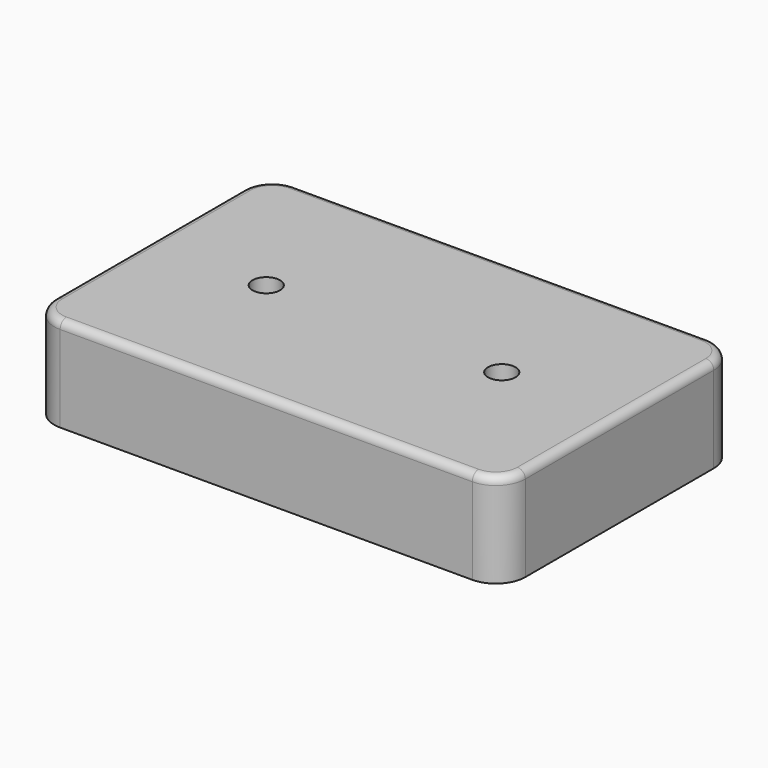
from build123d import *

# Parameters (mm, degrees)
F0_W         = 120
F0_H         = 75
F1_DEPTH     = 4
F2_W         = 120
F2_H         = 75
F3_DEPTH     = 20
F4_R         = 2
F5_T1_DEPTH  = 42.75
F5_T4_ANGLE  = 90
F5_T6_ANGLE  = 90
F5_T8_ANGLE  = 90
F5_T10_ANGLE = 90
F6_R         = 3.5
F7_DEPTH     = 25
F8_R         = 1.7577503979
F8_R_2       = 1.75
F9_DEPTH     = 10


# Not quite as in the source:
# - a fillet or chamfer that OpenCascade refuses, or shapes differently, is made with other operations: its cross-section is extruded or revolved along the edge and cut away or added


with BuildPart() as f1:
    # F0 (on Top) → F1 (new body)
    with BuildSketch(Plane.XY):
        Rectangle(F0_W, F0_H)
    extrude(amount=F1_DEPTH)

    # F2 (on face) → F3 (join)
    with BuildSketch(Plane(origin=(0, 0, 0), x_dir=(1, 0, 0), z_dir=(0, 0, -1))):
        Rectangle(F2_W, F2_H)
        Polygon((54.339364171, -27.5), (50, -27.5), (50, -31.3459709287), (-50, -31.3459709287), (-50, -27.5), (-54.5065030456, -27.5), (-54.5065030456, 27.5), (-50, 27.5), (-50, 32.2239883244), (50, 32.2239883244), (50, 27.5), (54.339364171, 27.5), align=None, mode=Mode.SUBTRACT)
    extrude(amount=F3_DEPTH)

    # F4
    f4_edges = [f1.edges().sort_by_distance(p)[0] for p in [
        (60, 0, 4),
        (0, -37.5, 4),
        (-60, 0, 4),
        (0, 37.5, 4),
    ]]
    fillet(f4_edges, radius=F4_R)

    # F5: fillet of radius 7.5 on 4 edges, made by hand

    # F5_s2 → F5_t1 (cut)
    with BuildSketch(Plane.XY.offset(-38.75)):
        with BuildLine():
            ThreePointArc((60, -30), (57.8033008589, -35.3033008589), (52.5, -37.5))
            Line((52.5, -37.5), (60, -37.5))
            Line((60, -37.5), (60, -30))
        make_face()
        with BuildLine():
            ThreePointArc((60, 30), (57.8033008589, 35.3033008589), (52.5, 37.5))
            Line((52.5, 37.5), (60, 37.5))
            Line((60, 37.5), (60, 30))
        make_face()
        with BuildLine():
            ThreePointArc((-52.5, -37.5), (-57.8033008589, -35.3033008589), (-60, -30))
            Line((-60, -30), (-60, -37.5))
            Line((-60, -37.5), (-52.5, -37.5))
        make_face()
        with BuildLine():
            ThreePointArc((-52.5, 37.5), (-57.8033008589, 35.3033008589), (-60, 30))
            Line((-60, 30), (-60, 37.5))
            Line((-60, 37.5), (-52.5, 37.5))
        make_face()
    extrude(amount=F5_T1_DEPTH, mode=Mode.SUBTRACT)

    # F5_s3 → F5_t4 (revolve, cut)
    with BuildSketch(Plane.YZ.offset(-52.5)):
        with BuildLine():
            ThreePointArc((35.5, 4), (36.9142135624, 3.4142135624), (37.5, 2))
            Line((37.5, 2), (37.5, 4))
            Line((37.5, 4), (35.5, 4))
        make_face()
    revolve(axis=Axis((-52.5, 30, 4), (0, 0, 1)), revolution_arc=F5_T4_ANGLE, mode=Mode.SUBTRACT)

    # F5_s5 → F5_t6 (revolve, cut)
    with BuildSketch(Plane.XZ.offset(30)):
        with BuildLine():
            ThreePointArc((-58, 4), (-59.4142135624, 3.4142135624), (-60, 2))
            Line((-60, 2), (-60, 4))
            Line((-60, 4), (-58, 4))
        make_face()
    revolve(axis=Axis((-52.5, -30, 4), (0, 0, 1)), revolution_arc=F5_T6_ANGLE, mode=Mode.SUBTRACT)

    # F5_s7 → F5_t8 (revolve, cut)
    with BuildSketch(Plane.XZ.offset(-30)):
        with BuildLine():
            ThreePointArc((58, 4), (59.4142135624, 3.4142135624), (60, 2))
            Line((60, 2), (60, 4))
            Line((60, 4), (58, 4))
        make_face()
    revolve(axis=Axis((52.5, 30, 4), (0, 0, 1)), revolution_arc=F5_T8_ANGLE, mode=Mode.SUBTRACT)

    # F5_s9 → F5_t10 (revolve, cut)
    with BuildSketch(Plane.YZ.offset(52.5)):
        with BuildLine():
            ThreePointArc((-35.5, 4), (-36.9142135624, 3.4142135624), (-37.5, 2))
            Line((-37.5, 2), (-37.5, 4))
            Line((-37.5, 4), (-35.5, 4))
        make_face()
    revolve(axis=Axis((52.5, -30, 4), (0, 0, 1)), revolution_arc=F5_T10_ANGLE, mode=Mode.SUBTRACT)

    # F6 (on face) → F7 (cut)
    with BuildSketch(Plane.XY.offset(4)):
        with Locations((-30, 0)):
            Circle(F6_R)
        with Locations((30, 0)):
            Circle(F6_R)
    extrude(amount=-F7_DEPTH, mode=Mode.SUBTRACT)

    # F8 (on face) → F9 (cut)
    with BuildSketch(Plane(origin=(0, 0, -20), x_dir=(1, 0, 0), z_dir=(0, 0, -1))):
        with Locations((-54.5065030456, 32.2239883244)):
            Circle(F8_R)
        with Locations((54.339364171, 32.2239883244)):
            Circle(F8_R_2)
        with Locations((54.339364171, -31.3459709287)):
            Circle(F8_R_2)
        with Locations((-54.5065030456, -31.3459709287)):
            Circle(F8_R_2)
    extrude(amount=-F9_DEPTH, mode=Mode.SUBTRACT)


solid = f1.part
